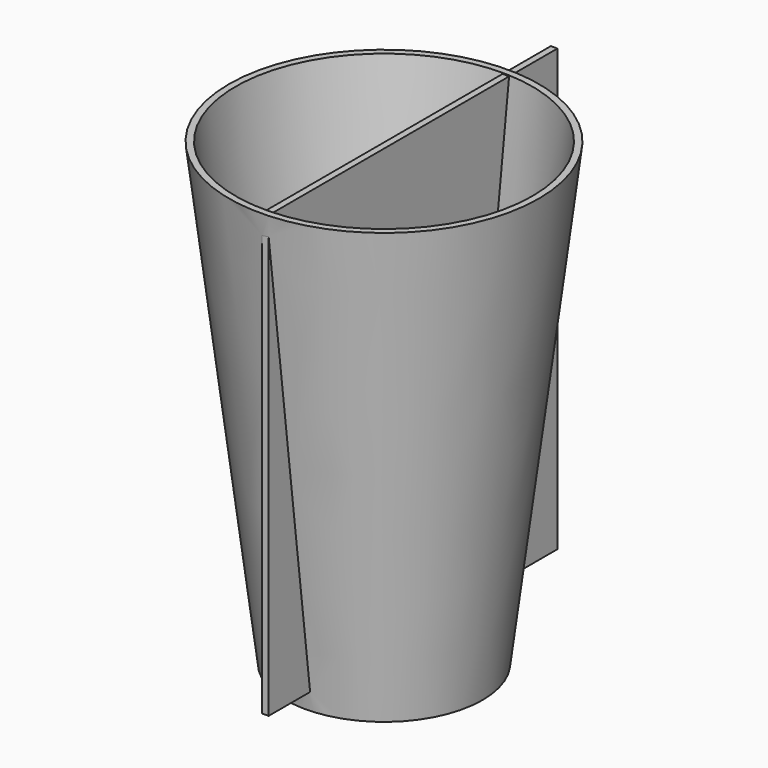
from build123d import *

# Parameters (mm, degrees)
F0_R     = 38.1
F1_DEPTH = 177.8
F1_TAPER = -7
F2_T     = -2.54
F3_W     = 139.5735256374
F3_H     = 170.4298052937
F4_DEPTH = 2.54


# Not quite as in the source:
# - a feature names something its author has since deleted; it is built from what else it names


with BuildPart() as f1:
    # F0 (on Top) → F1 (new body)
    with BuildSketch(Plane.XY):
        Circle(F0_R)
    extrude(amount=F1_DEPTH, taper=F1_TAPER)

    # F2
    f2_openings = [f1.faces().sort_by_distance(p)[0] for p in [
        (0, 0, 177.8),
    ]]
    offset(amount=F2_T, openings=f2_openings, kind=Kind.INTERSECTION)

    # F3 (on Right) → F4 (join)
    with BuildSketch(Plane.YZ):
        with Locations((10.8456704766, 92.2188116238)):
            Rectangle(F3_W, F3_H)
    extrude(amount=F4_DEPTH)


solid = f1.part
